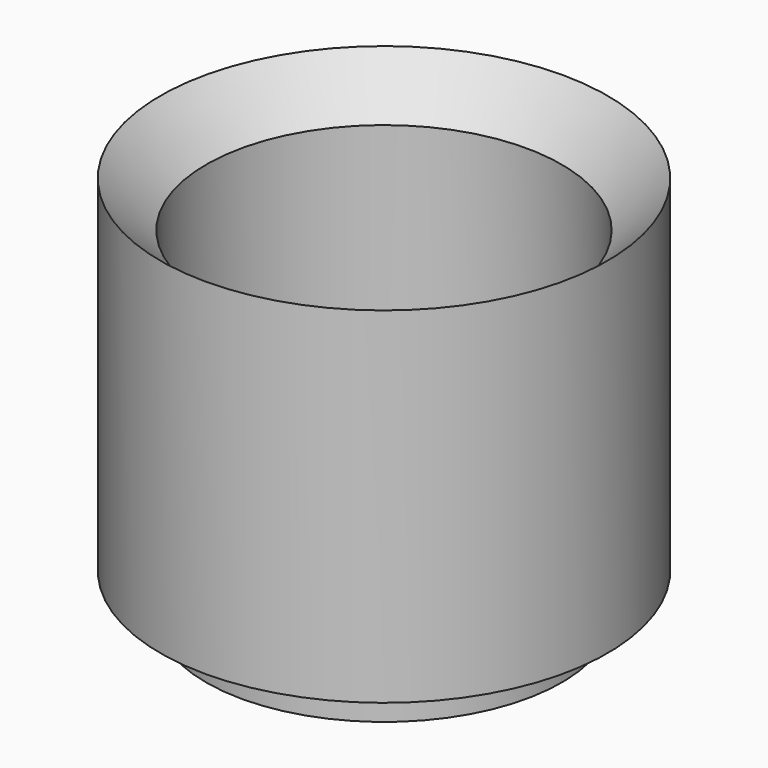
from build123d import *

# Parameters (mm, degrees)
F2_SIZE = 8.99999


# Not quite as in the source:
# - a fillet or chamfer is up to 0.001 mm smaller than in the source, because OpenCascade refuses the exact size


with BuildPart() as f1:
    # F0 (on Right) → F1 (revolve)
    with BuildSketch(Plane.YZ):
        Polygon((-37.8479540345, 16.603627705), (-37.8479540345, 76.603627705), (-46.8479540345, 76.603627705), (-46.8479540345, 8.603627705), (-37.8479540345, 8.603627705), (-37.8479540345, 0.603627705), (-2.8479540345, 0.603627705), (-2.8479540345, 8.603627705), (-27.8479540345, 8.603627705), (-27.8479540345, 16.603627705), align=None)
    revolve(axis=Axis((0, -2.8479540345, 4.603627705), (0, 0, 1)))

    # F2 (size 9 in the source; OpenCascade refuses exactly that, so slightly less here)
    f2_edges = [f1.edges().sort_by_distance(p)[0] for p in [
        (0, 32.152046, 76.603628),
    ]]
    chamfer(f2_edges, length=F2_SIZE)


solid = f1.part
